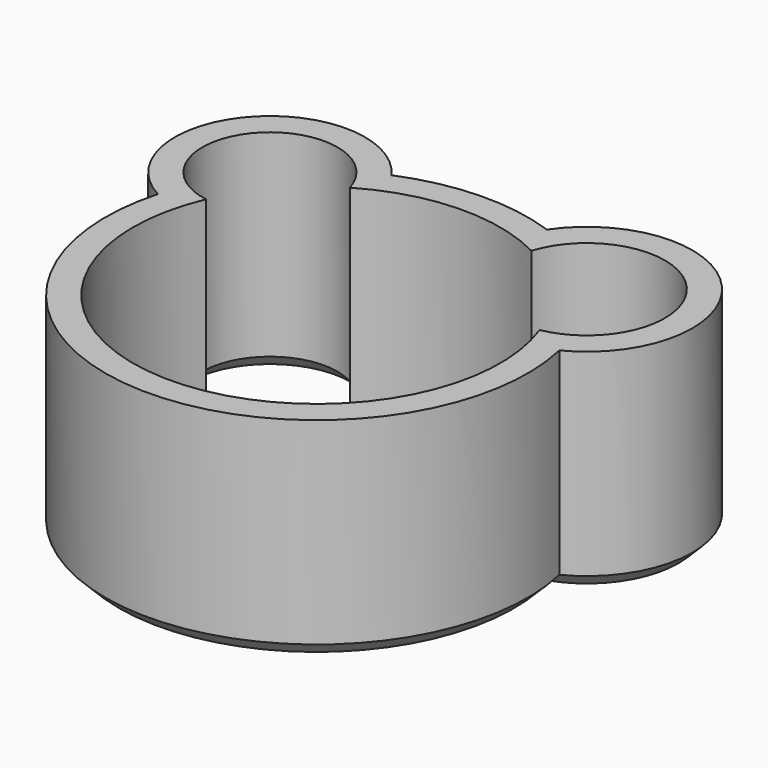
from build123d import *

# Parameters (mm, degrees)
F1_DEPTH = 25.4
F2_SIZE  = 1.65099


# Not quite as in the source:
# - a fillet or chamfer is up to 0.001 mm smaller than in the source, because OpenCascade refuses the exact size


with BuildPart() as f1:
    # F0 (on Top) → F1 (new body)
    with BuildSketch(Plane.XY):
        with BuildLine():
            ThreePointArc((24.8022671705, 5.4779141289), (28.575, 25.2007812379), (8.5352328295, 23.9229973153))
            ThreePointArc((8.5352328295, 23.9229973153), (-0.6536534353, 25.3915879217), (-9.754807335, 23.4521584051))
            ThreePointArc((-9.754807335, 23.4521584051), (-27.6224996448, 24.3607548834), (-24.4875679847, 6.7467780603))
            ThreePointArc((-24.4875679847, 6.7467780603), (-0.6536534353, -25.3915879217), (24.8022671705, 5.4779141289))
        make_face()
        with BuildLine():
            ThreePointArc((-20.2845825482, 8.7668303761), (-25.1459996448, 22.1766871761), (-11.2336426791, 19.0296315298))
            ThreePointArc((-11.2336426791, 19.0296315298), (-0.6492677951, 22.0884597772), (10.0965, 19.6566093656))
            ThreePointArc((10.0965, 19.6566093656), (26.0985, 23.0167135306), (20.7645, 7.5602343714))
            ThreePointArc((20.7645, 7.5602343714), (-0.6492677951, -22.0884597772), (-20.2845825482, 8.7668303761))
        make_face(mode=Mode.SUBTRACT)
    extrude(amount=F1_DEPTH)

    # F2 (size 1.651 in the source; OpenCascade refuses exactly that, so slightly less here)
    f2_edges = [f1.edges().sort_by_distance(p)[0] for p in [
        (-0.653653, -25.391588, 0),
        (-0.649268, -22.08846, 0),
        (-25.146, 22.176687, 0),
        (-27.6225, 24.360755, 0),
        (-0.649268, 22.08846, 0),
        (-0.653653, 25.391588, 0),
        (28.575, 25.200781, 0),
        (26.0985, 23.016714, 0),
    ]]
    chamfer(f2_edges, length=F2_SIZE)


solid = f1.part
